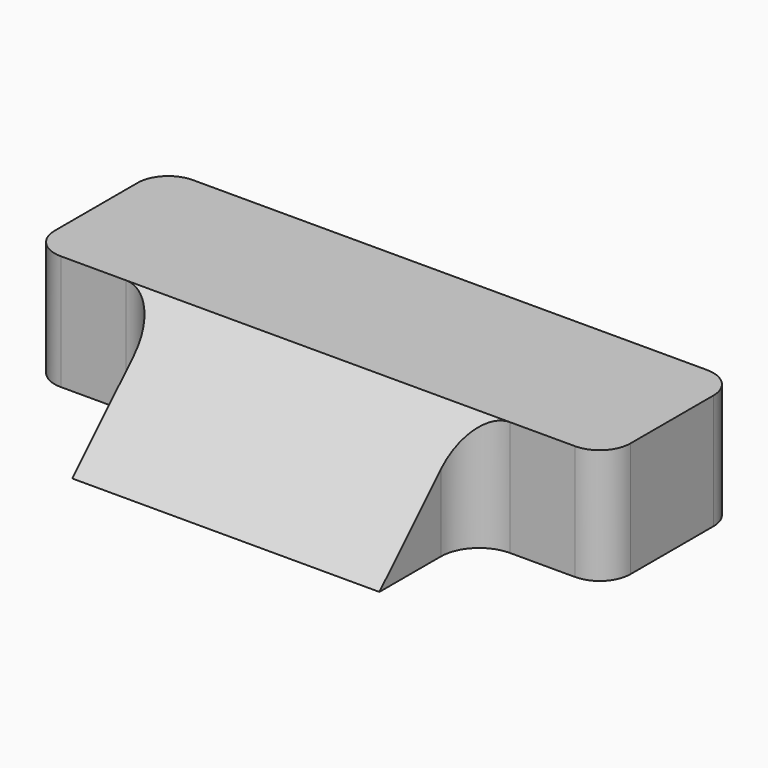
from build123d import *

# Parameters (mm, degrees)
F0_W      = 190.5
F0_H      = 54.61
F1_DEPTH  = 38.1
F2_W      = 165.1
F2_H      = 29.21
F3_DEPTH  = 25.4
F4_W      = 101.6
F4_H      = 38.1
F5_DEPTH  = 38.1
F6_SIZE   = 38.09999
F7_R      = 10.16
F8_R      = 10.16
F9_W      = 101.6
F9_H      = 38.1
F10_DEPTH = 38.1
F11_SIZE  = 38.09999
F12_R     = 12.7


# Not quite as in the source:
# - a fillet or chamfer is up to 0.001 mm smaller than in the source, because OpenCascade refuses the exact size


with BuildPart() as f1:
    # F0 (on Top) → F1 (new body)
    with BuildSketch(Plane.XY):
        Rectangle(F0_W, F0_H)
    extrude(amount=F1_DEPTH)

    # F2 (on face) → F3 (cut)
    with BuildSketch(Plane(origin=(0, 0, 0), x_dir=(1, 0, 0), z_dir=(0, 0, -1))):
        Rectangle(F2_W, F2_H)
    extrude(amount=-F3_DEPTH, mode=Mode.SUBTRACT)

    # F4 (on face) → F5 (join)
    with BuildSketch(Plane(origin=(0, 27.305, 0), x_dir=(-1, 0, 0), z_dir=(0, 1, 0))):
        with Locations((0, 19.05)):
            Rectangle(F4_W, F4_H)
    extrude(amount=F5_DEPTH)

    # F6 (size 38.1 in the source; OpenCascade refuses exactly that, so slightly less here)
    f6_edges = [f1.edges().sort_by_distance(p)[0] for p in [
        (0, 65.405, 38.1),
    ]]
    chamfer(f6_edges, length=F6_SIZE)

    # F7 (call 1 of 2: OpenCascade refuses the feature's edges together)
    f7_edges = [f1.edges().sort_by_distance(p)[0] for p in [
        (-50.8, 27.305, 19.05),
    ]]
    fillet(f7_edges, radius=F7_R)

    # F7#2 (call 2 of 2)
    f7_2_edges = [f1.edges().sort_by_distance(p)[0] for p in [
        (50.8, 27.305, 19.05),
    ]]
    fillet(f7_2_edges, radius=F7_R)

    # F8
    f8_edges = [f1.edges().sort_by_distance(p)[0] for p in [
        (-95.25, 27.305, 19.05),
        (-95.25, -27.305, 19.05),
        (95.25, 27.305, 19.05),
        (95.25, -27.305, 19.05),
    ]]
    fillet(f8_edges, radius=F8_R)

    # F9 (on face) → F10 (join)
    with BuildSketch(Plane.XZ.offset(27.305)):
        with Locations((0, 19.05)):
            Rectangle(F9_W, F9_H)
    extrude(amount=F10_DEPTH)

    # F11 (size 38.1 in the source; OpenCascade refuses exactly that, so slightly less here)
    f11_edges = [f1.edges().sort_by_distance(p)[0] for p in [
        (0, -65.405, 38.1),
    ]]
    chamfer(f11_edges, length=F11_SIZE)

    # F12 (call 1 of 2: OpenCascade refuses the feature's edges together)
    f12_edges = [f1.edges().sort_by_distance(p)[0] for p in [
        (50.8, -27.305, 19.05),
    ]]
    fillet(f12_edges, radius=F12_R)

    # F12#2 (call 2 of 2)
    f12_2_edges = [f1.edges().sort_by_distance(p)[0] for p in [
        (-50.8, -27.305, 19.05),
    ]]
    fillet(f12_2_edges, radius=F12_R)


solid = f1.part
